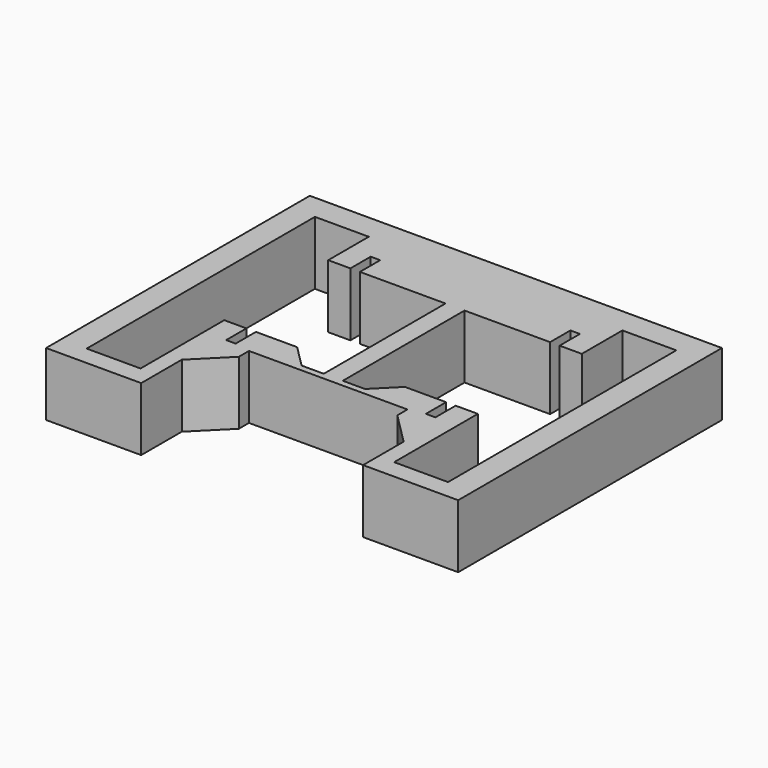
from build123d import *

# Parameters (mm, degrees)
F1_DEPTH  = 20
F2_DEPTH  = 12
F3_DEPTH  = 10
F4_DEPTH  = 10
F5_W      = 25
F5_H      = 20
F6_DEPTH  = 14
F7_SIZE   = 10
F8_SIZE   = 6.99999
F9_DEPTH  = 10
F10_W     = 17
F10_H     = 80
F11_DEPTH = 20.001
F13_DEPTH = 20


# Not quite as in the source:
# - a fillet or chamfer is up to 0.001 mm smaller than in the source, because OpenCascade refuses the exact size
# - a feature names something its author has since deleted; it is built from what else it names


with BuildPart() as f1:
    # F0 (on Top) → F1 (new body)
    with BuildSketch(Plane.XY):
        Polygon((78, -43.2), (75, -45), (78, -45), align=None)
        Polygon((33.3333333333, -20), (0, 0), (0, -90), (33.3333333333, -70), (25, -70), (25, -20), align=None)
        Polygon((150, -90), (150, 0), (116.6666666667, -20), (125, -20), (125, -70), (116.6666666667, -70), align=None)
        Polygon((75, 0), (0, 0), (33.3333333333, -20), (35, -20), (35, -14), (42, -14), (42, -6), (45, -6), (45, -14), (72, -14), (72, -43.2), (75, -45), align=None)
        Polygon((150, 0), (75, 0), (75, -45), (78, -43.2), (78, -14), (105, -14), (105, -6), (108, -6), (108, -14), (115, -14), (115, -20), (116.6666666667, -20), align=None)
        Polygon((78, -45), (75, -45), (78, -46.8), align=None)
        Polygon((72, -45), (75, -45), (72, -43.2), align=None)
        Polygon((72, -46.8), (75, -45), (72, -45), align=None)
        Polygon((78, -46.8), (75, -45), (75, -90), (150, -90), (116.6666666667, -70), (115, -70), (115, -69), (105, -63), (91.6666666667, -55), (85, -55), (85, -62), (78, -62), (78, -55), (78, -48), align=None)
        Polygon((33.3333333333, -70), (0, -90), (75, -90), (75, -45), (72, -46.8), (72, -48), (72, -55), (72, -62), (65, -62), (65, -55), (58.3333333333, -55), (45, -63), (35, -69), (35, -70), align=None)
        Polygon((35, -55), (35, -69), (45, -63), (42, -63), (42, -55), align=None)
        Polygon((45, -63), (58.3333333333, -55), (45, -55), align=None)
        Polygon((105, -55), (91.6666666667, -55), (105, -63), align=None)
        Polygon((105, -63), (115, -69), (115, -55), (108, -55), (108, -63), align=None)
    extrude(amount=F1_DEPTH)

    # F2 (cut): a face of the model
    f2_faces = [f1.faces().sort_by_distance(p)[0] for p in [
        (75, -90, 10),
    ]]
    extrude(f2_faces, amount=-F2_DEPTH, mode=Mode.SUBTRACT)

    # F3 (cut): a face of the model
    f3_faces = [f1.faces().sort_by_distance(p)[0] for p in [
        (150, -39, 10),
    ]]
    extrude(f3_faces, amount=-F3_DEPTH, mode=Mode.SUBTRACT)

    # F4 (cut): a face of the model
    f4_faces = [f1.faces().sort_by_distance(p)[0] for p in [
        (0, -39, 10),
    ]]
    extrude(f4_faces, amount=-F4_DEPTH, mode=Mode.SUBTRACT)

    # F5 (on face) → F6 (cut)
    with BuildSketch(Plane.XZ.offset(78)):
        with Locations((87.5, 10)):
            Rectangle(F5_W, F5_H)
        with Locations((62.5, 10)):
            Rectangle(F5_W, F5_H)
    extrude(amount=-F6_DEPTH, mode=Mode.SUBTRACT)

    # F7
    f7_edges = [f1.edges().sort_by_distance(p)[0] for p in [
        (100, -78, 10),
        (50, -78, 10),
    ]]
    chamfer(f7_edges, length=F7_SIZE)

    # F8 (size 7 in the source; OpenCascade refuses exactly that, so slightly less here)
    f8_edges = [f1.edges().sort_by_distance(p)[0] for p in [
        (85, -55, 10),
        (65, -55, 10),
    ]]
    chamfer(f8_edges, length=F8_SIZE)

    # F9 (add): a face of the model
    f9_faces = [f1.faces().sort_by_distance(p)[0] for p in [
        (75, 0, 10),
    ]]
    extrude(f9_faces, amount=F9_DEPTH)

    # F10 (on face) → F11 (cut, through all)
    with BuildSketch(Plane.XY.offset(20)):
        with Locations((26.5, -38)):
            Rectangle(F10_W, F10_H)
        with Locations((123.5, -38)):
            Rectangle(F10_W, F10_H)
    extrude(amount=-F11_DEPTH, mode=Mode.SUBTRACT)

    # F12 (on face) → F13 (join)
    with BuildSketch(Plane.XY.offset(20)):
        Polygon((18, -88), (18, -78), (10, -78), (10, -94), (40, -94), (40, -78), (35, -78), (35, -88), align=None)
        Polygon((140, -94), (140, -78), (132, -78), (132, -88), (115, -88), (115, -78), (110, -78), (110, -94), align=None)
    extrude(amount=-F13_DEPTH)


solid = f1.part
